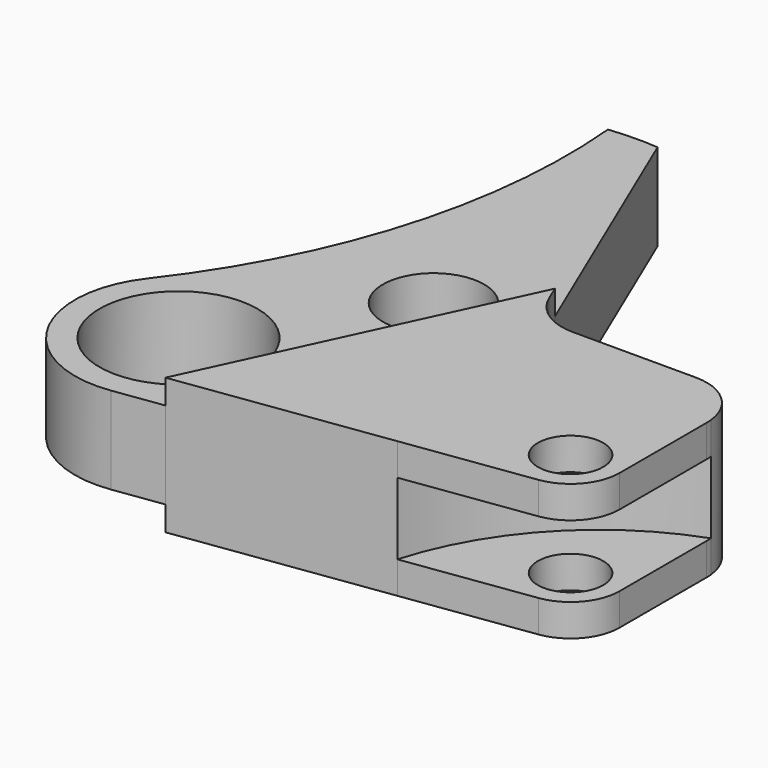
from build123d import *

# Parameters (mm, degrees)
F0_R     = 14.5
F0_R_2   = 9.3
F1_DEPTH = 8
F2_DEPTH = 12.5
F0_R_3   = 6
F3_DEPTH = 6.6
F4_DEPTH = 5.9
F5_DEPTH = 5.9


with BuildPart() as f1:
    # F0 (on Top) → F1 (new body, symmetric)
    with BuildSketch(Plane.XY):
        with BuildLine():
            Line((2.6379834818, -18.8137083294), (11.6484677091, -17.5502940073))
            Line((11.6484677091, -17.5502940073), (37.9808631577, 38.9197102657))
            Line((37.9808631577, 38.9197102657), (16.6523997132, 89.1664213307))
            ThreePointArc((16.6523997132, 89.1664213307), (12.1489449291, 89.292756528), (7.6523997132, 89.0132092222))
            ThreePointArc((7.6523997132, 89.0132092222), (3.6651197911, 48.1806616582), (-15.0070128486, 11.6492121327))
            ThreePointArc((-15.0070128486, 11.6492121327), (-16.4391484767, -9.5220257988), (2.6379834818, -18.8137083294))
        make_face()
        Circle(F0_R, mode=Mode.SUBTRACT)
        with Locations((21.8, 31.3)):
            Circle(F0_R_2, mode=Mode.SUBTRACT)
    extrude(amount=F1_DEPTH, both=True)

    # F0 (on Top) → F2 (join, symmetric)
    with BuildSketch(Plane.XY):
        with BuildLine():
            Line((11.6484677091, -17.5502940073), (49.9478345026, -12.1801088639))
            ThreePointArc((49.9478345026, -12.1801088639), (61.4641714079, 8.1340479446), (80.9495714617, 21.0030093362))
            ThreePointArc((80.9495714617, 21.0030093362), (77.7070823253, 27.4172128648), (71, 30))
            Line((71, 30), (48.3859111453, 30))
            ThreePointArc((48.3859111453, 30), (42.8665412922, 31.6611417793), (39.1808626108, 36.0926887151))
            Line((39.1808626108, 36.0926887151), (37.9808631577, 38.9197102657))
            Line((37.9808631577, 38.9197102657), (11.6484677091, -17.5502940073))
        make_face()
    extrude(amount=F2_DEPTH, both=True)



with BuildPart() as f3:
    # F0 (on Top) → F3 (new body, symmetric)
    with BuildSketch(Plane.XY):
        with BuildLine():
            Line((49.9478345026, -12.1801088639), (73.2497189898, -8.9128111416))
            ThreePointArc((73.2497189898, -8.9128111416), (78.7914457558, -5.9056129695), (81, 0))
            Line((81, 0), (81, 20))
            ThreePointArc((81, 20), (80.9873849084, 20.5021381199), (80.9495714617, 21.0030093362))
            ThreePointArc((80.9495714617, 21.0030093362), (61.4641714079, 8.1340479446), (49.9478345026, -12.1801088639))
        make_face()
        with Locations((72, 0)):
            Circle(F0_R_3, mode=Mode.SUBTRACT)
    extrude(amount=F3_DEPTH, both=True)


with BuildPart() as f1_1:
    add(f1.part)
    # F4 (add, through all): a face of the model
    f4_faces = [f3.part.faces().sort_by_distance(p)[0] for p in [
        (61.7962542599, 7.8237954492, 6.6),
    ]]
    extrude(f4_faces, amount=F4_DEPTH)

    # F5 (add, through all): a face of the model
    f5_faces = [f3.part.faces().sort_by_distance(p)[0] for p in [
        (61.7962542599, 7.8237954492, -6.6),
    ]]
    extrude(f5_faces, amount=F5_DEPTH)

    # F6: cut F3
    add(f3.part, mode=Mode.SUBTRACT)


solid = f1_1.part
